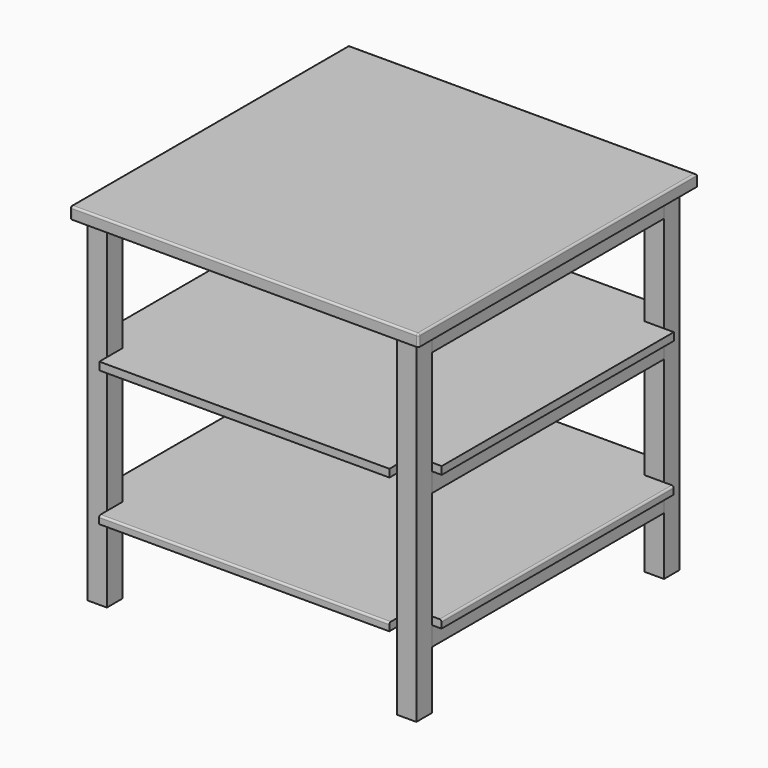
from build123d import *

# Parameters (mm, degrees)
F0_W      = 50
F0_H      = 50
F1_DEPTH  = 870
F4_W      = 900
F4_H      = 900
F5_DEPTH  = 30
F8_DEPTH  = 20
F9_R      = 5
F10_R     = 5
F11_R     = 5
F3_W      = 50
F3_H      = 50
F12_DEPTH = 750
F14_DEPTH = 20


with BuildPart() as f1:
    # F0 (on Top) → F1 (new body)
    with BuildSketch(Plane.XY):
        with Locations((-47.9233672377, -781.426829705)):
            Rectangle(F0_W, F0_H)
    extrude(amount=-F1_DEPTH)


with BuildPart() as f1b:
    # F0 (on Top) → F1, piece 2 (new body)
    with BuildSketch(Plane.XY):
        with Locations((-47.9233672377, 18.573170295)):
            Rectangle(F0_W, F0_H)
    extrude(amount=-F1_DEPTH)


with BuildPart() as f1c:
    # F0 (on Top) → F1, piece 3 (new body)
    with BuildSketch(Plane.XY):
        with Locations((752.0766327623, -781.426829705)):
            Rectangle(F0_W, F0_H)
    extrude(amount=-F1_DEPTH)


with BuildPart() as f1d:
    # F0 (on Top) → F1, piece 4 (new body)
    with BuildSketch(Plane.XY):
        with Locations((752.0766327623, 18.573170295)):
            Rectangle(F0_W, F0_H)
    extrude(amount=-F1_DEPTH)


with BuildPart() as f5:
    # F4 (on face) → F5 (new body)
    with BuildSketch(Plane.XY):
        with Locations((352.0766327623, -381.426829705)):
            Rectangle(F4_W, F4_H)
    extrude(amount=F5_DEPTH)

    # F9
    f9_edges = [f5.edges().sort_by_distance(p)[0] for p in [
        (352.076633, -831.42683, 30),
    ]]
    fillet(f9_edges, radius=F9_R)

    # F10
    f10_edges = [f5.edges().sort_by_distance(p)[0] for p in [
        (802.076633, -378.92683, 30),
        (-97.923367, -378.92683, 30),
        (352.076633, 68.57317, 30),
    ]]
    fillet(f10_edges, radius=F10_R)


with BuildPart() as f8:
    # F7 (on face) → F8 (new body)
    with BuildSketch(Plane.XY.offset(-670)):
        Polygon((727.0766327623, -756.426829705), (802.0766327623, -756.426829705), (802.0766327623, -6.426829705), (727.0766327623, -6.426829705), (727.0766327623, 68.573170295), (-22.9233672377, 68.573170295), (-22.9233672377, -6.426829705), (-97.9233672377, -6.426829705), (-97.9233672377, -756.426829705), (-22.9233672377, -756.426829705), (-22.9233672377, -831.426829705), (727.0766327623, -831.426829705), align=None)
    extrude(amount=F8_DEPTH)

    # F11
    f11_edges = [f8.edges().sort_by_distance(p)[0] for p in [
        (802.076633, -381.42683, -650),
        (352.076633, 68.57317, -650),
        (352.076633, -831.42683, -650),
        (-97.923367, -381.42683, -650),
    ]]
    fillet(f11_edges, radius=F11_R)


with BuildPart() as f12:
    # F3 (on face) → F12 (new body)
    with BuildSketch(Plane(origin=(0, -756.426829705, 0), x_dir=(-1, 0, 0), z_dir=(0, 1, 0))):
        with Locations((-752.0766327623, -695)):
            Rectangle(F3_W, F3_H)
    extrude(amount=F12_DEPTH)


with BuildPart() as f12b:
    # F3 (on face) → F12, piece 2 (new body)
    with BuildSketch(Plane(origin=(0, -756.426829705, 0), x_dir=(-1, 0, 0), z_dir=(0, 1, 0))):
        with Locations((47.9233672377, -695)):
            Rectangle(F3_W, F3_H)
    extrude(amount=F12_DEPTH)


with BuildPart() as f12c:
    # F3 (on face) → F12, piece 3 (new body)
    with BuildSketch(Plane(origin=(0, -756.426829705, 0), x_dir=(-1, 0, 0), z_dir=(0, 1, 0))):
        with Locations((47.9233672377, -25)):
            Rectangle(F3_W, F3_H)
    extrude(amount=F12_DEPTH)


with BuildPart() as f12d:
    # F3 (on face) → F12, piece 4 (new body)
    with BuildSketch(Plane(origin=(0, -756.426829705, 0), x_dir=(-1, 0, 0), z_dir=(0, 1, 0))):
        with Locations((-752.0766327623, -25)):
            Rectangle(F3_W, F3_H)
    extrude(amount=F12_DEPTH)


with BuildPart() as f12e:
    # F3 (on face) → F12, piece 5 (new body)
    with BuildSketch(Plane(origin=(0, -756.426829705, 0), x_dir=(-1, 0, 0), z_dir=(0, 1, 0))):
        with Locations((47.9233672377, -345)):
            Rectangle(F3_W, F3_H)
    extrude(amount=F12_DEPTH)


with BuildPart() as f12f:
    # F3 (on face) → F12, piece 6 (new body)
    with BuildSketch(Plane(origin=(0, -756.426829705, 0), x_dir=(-1, 0, 0), z_dir=(0, 1, 0))):
        with Locations((-752.0766327623, -345)):
            Rectangle(F3_W, F3_H)
    extrude(amount=F12_DEPTH)


with BuildPart() as f14:
    # F13 (on face) → F14 (new body)
    with BuildSketch(Plane.XY.offset(-320)):
        Polygon((727.49376297, -756.4368884079), (802.49376297, -756.4368884079), (802.49376297, -6.4368884079), (727.49376297, -6.4368884079), (727.49376297, 68.5631115921), (-22.50623703, 68.5631115921), (-22.50623703, -6.4368884079), (-97.50623703, -6.4368884079), (-97.50623703, -756.4368884079), (-22.50623703, -756.4368884079), (-22.50623703, -831.4368884079), (727.49376297, -831.4368884079), align=None)
    extrude(amount=F14_DEPTH)


solid = Compound([f1.part, f1b.part, f1c.part, f1d.part, f5.part, f8.part, f12.part, f12b.part, f12c.part, f12d.part, f12e.part, f12f.part, f14.part])
